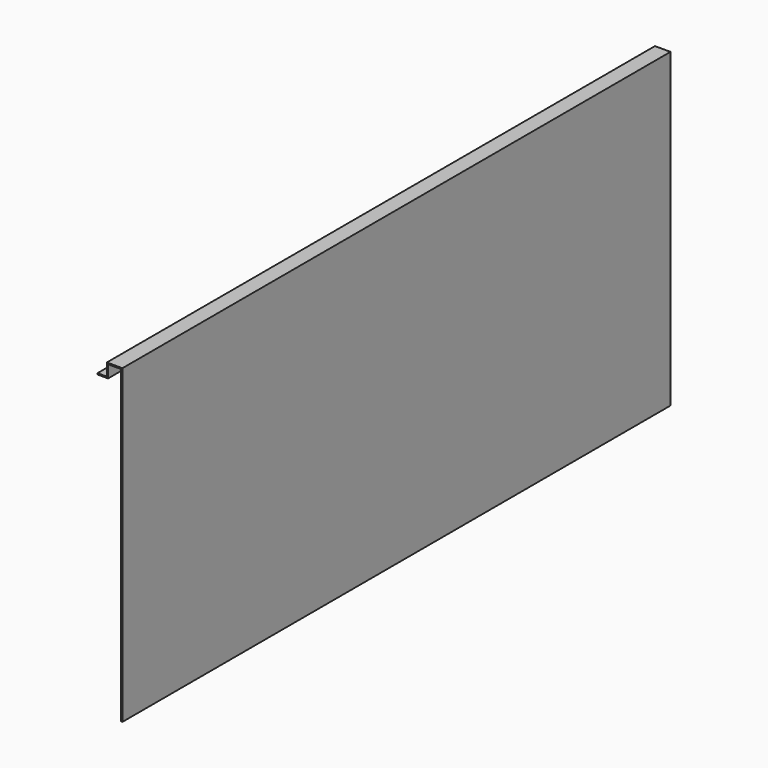
from build123d import *

# Parameters (mm, degrees)
F1_DEPTH = 1100


# Not quite as in the source:
# - a feature names something its author has since deleted; it is built from what else it names


with BuildPart() as f1:
    # F0 (on Front) → F1 (new body)
    with BuildSketch(Plane.XZ):
        Polygon((-15.4624978453, 35.3617481887), (-30.4624978453, 35.3617481887), (-30.4624978453, 33.3617481887), (-13.4624978453, 33.3617481887), (-13.4624978453, 53.3617481887), (7.5375021547, 53.3617481887), (7.5375021547, -444.6382518113), (9.5375021547, -444.6382518113), (9.5375021547, 55.3617481887), (-15.4624978453, 55.3617481887), align=None)
    extrude(amount=F1_DEPTH)


solid = f1.part
